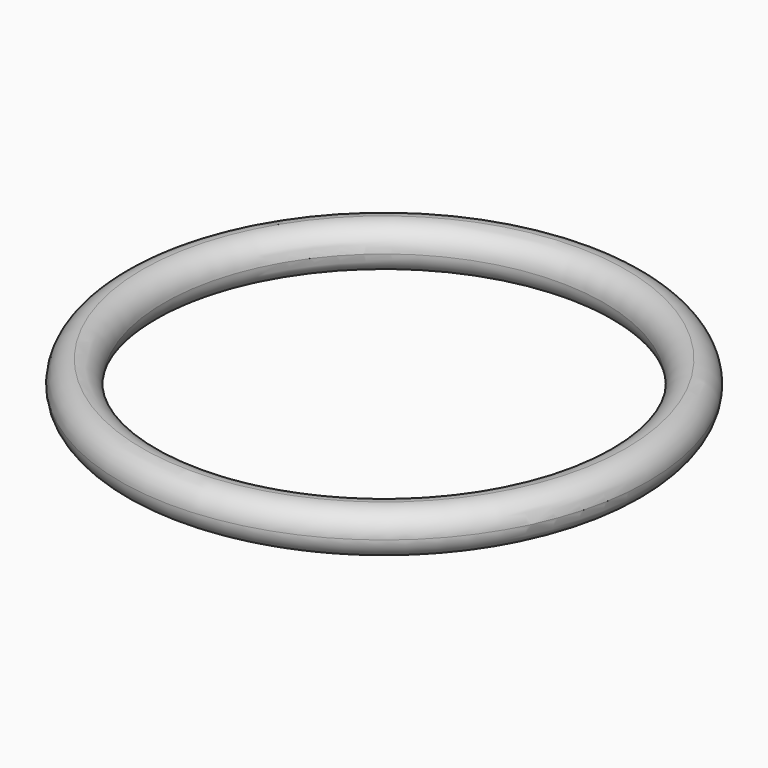
from build123d import *

# Parameters (mm, degrees)
F0_R     = 60
F0_R_2   = 50
F1_DEPTH = 10
F2_R     = 4.99999


# Not quite as in the source:
# - a fillet or chamfer is up to 0.001 mm smaller than in the source, because OpenCascade refuses the exact size


with BuildPart() as f1:
    # F0 (on Top) → F1 (new body)
    with BuildSketch(Plane.XY):
        with Locations((-48.8860793412, 39.2916202545)):
            Circle(F0_R)
        with Locations((-48.8860793412, 39.2916202545)):
            Circle(F0_R_2, mode=Mode.SUBTRACT)
    extrude(amount=F1_DEPTH)

    # F2 (radius 5 in the source; OpenCascade refuses exactly that, so slightly less here)
    f2_edges = [f1.edges().sort_by_distance(p)[0] for p in [
        (-108.886079, 39.29162, 10),
        (-108.886079, 39.29162, 0),
        (-98.886079, 39.29162, 10),
        (-98.886079, 39.29162, 0),
    ]]
    fillet(f2_edges, radius=F2_R)


solid = f1.part
